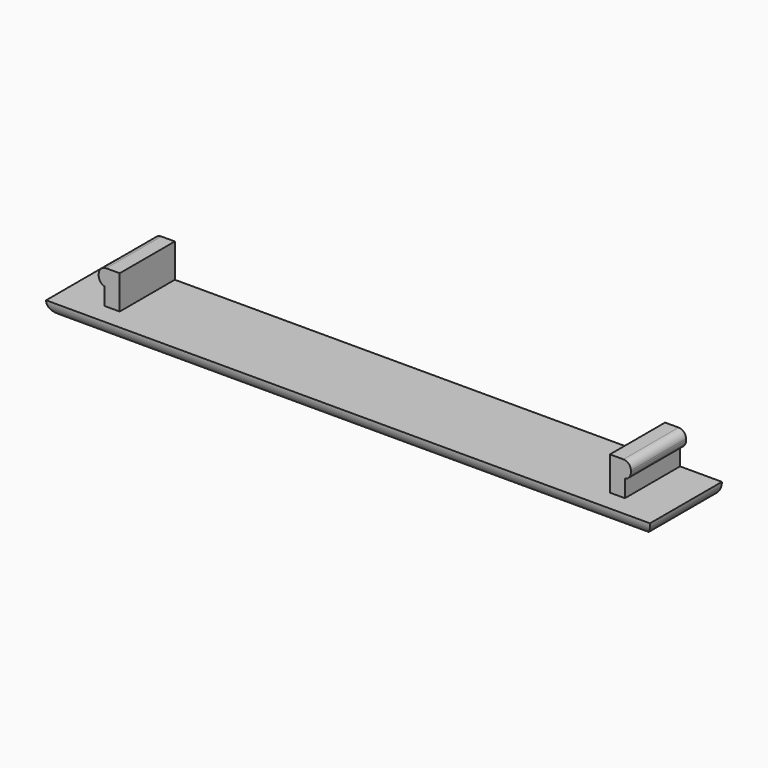
from build123d import *

# Parameters (mm, degrees)
F0_W        = 80.6
F0_H        = 12
F1_DEPTH    = 2
F2_W        = 2
F2_H        = 9.2
F3_DEPTH    = 4.5
F4_W        = 9.2
F4_H        = 2.2
F5_DEPTH    = 0.8
F6_R        = 1.99999
F7_W        = 9.2
F7_H        = 2.2
F8_DEPTH    = 0.8
F9_T1_DEPTH = 14.0989794856
F9_T3_DEPTH = 14.2


# Not quite as in the source:
# - a fillet or chamfer that OpenCascade refuses, or shapes differently, is made with other operations: its cross-section is extruded or revolved along the edge and cut away or added
# - a fillet or chamfer is up to 0.001 mm smaller than in the source, because OpenCascade refuses the exact size


with BuildPart() as f1:
    # F0 (on Top) → F1 (new body)
    with BuildSketch(Plane.XY):
        with Locations((-40.3, 6)):
            Rectangle(F0_W, F0_H)
    extrude(amount=-F1_DEPTH)

    # F2 (on face) → F3 (join)
    with BuildSketch(Plane.XY):
        with Locations((-74.015, 7.4)):
            Rectangle(F2_W, F2_H)
        with Locations((-6.585, 7.4)):
            Rectangle(F2_W, F2_H)
    extrude(amount=F3_DEPTH)

    # F4 (on face) → F5 (join)
    with BuildSketch(Plane(origin=(-75.015, 0, 0), x_dir=(0, -1, 0), z_dir=(-1, 0, 0))):
        with Locations((-7.4, 3.4)):
            Rectangle(F4_W, F4_H)
    extrude(amount=F5_DEPTH)

    # F6 (radius 2 in the source; OpenCascade refuses exactly that, so slightly less here)
    f6_edges = [f1.edges().sort_by_distance(p)[0] for p in [
        (-80.6, 6, -2),
        (0, 6, -2),
        (-40.3, 0, -2),
    ]]
    fillet(f6_edges, radius=F6_R)

    # F7 (on face) → F8 (join)
    with BuildSketch(Plane.YZ.offset(-5.585)):
        with Locations((7.4, 3.4)):
            Rectangle(F7_W, F7_H)
    extrude(amount=F8_DEPTH)

    # F9: fillet of radius 1 on 4 edges, made by hand

    # F9_s2 → F9_t1 (cut)
    with BuildSketch(Plane.XZ.offset(-14.4494897428)):
        with BuildLine():
            ThreePointArc((-5.585, 2.3), (-5.0104033308, 2.6473403651), (-4.785, 3.2797958971))
            Line((-4.785, 3.2797958971), (-4.785, 2.3))
            Line((-4.785, 2.3), (-5.585, 2.3))
        make_face()
        with BuildLine():
            ThreePointArc((-75.815, 3.2797958971), (-75.5895966692, 2.6473403651), (-75.015, 2.3))
            Line((-75.015, 2.3), (-75.815, 2.3))
            Line((-75.815, 2.3), (-75.815, 3.2797958971))
        make_face()
    extrude(amount=F9_T1_DEPTH, mode=Mode.SUBTRACT)

    # F9_s4 → F9_t3 (cut)
    with BuildSketch(Plane.XZ.offset(-14.5)):
        with BuildLine():
            ThreePointArc((-4.785, 3.5), (-5.0778932188, 4.2071067812), (-5.785, 4.5))
            Line((-5.785, 4.5), (-4.785, 4.5))
            Line((-4.785, 4.5), (-4.785, 3.5))
        make_face()
        with BuildLine():
            ThreePointArc((-74.815, 4.5), (-75.5221067812, 4.2071067812), (-75.815, 3.5))
            Line((-75.815, 3.5), (-75.815, 4.5))
            Line((-75.815, 4.5), (-74.815, 4.5))
        make_face()
    extrude(amount=F9_T3_DEPTH, mode=Mode.SUBTRACT)


solid = f1.part
